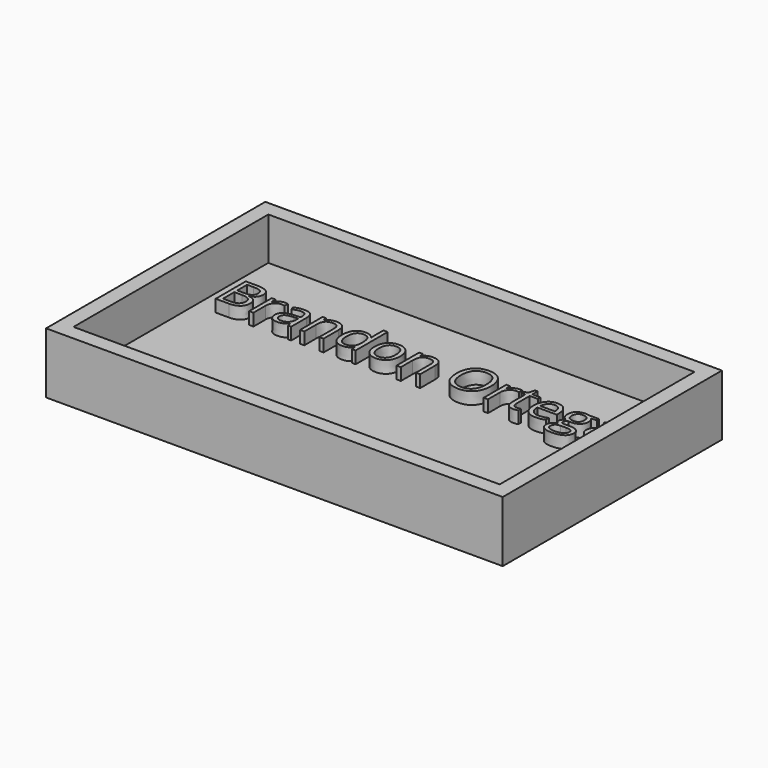
from build123d import *

# Parameters (mm, degrees)
F0_W         = 177.8
F0_H         = 101.6
F1_DEPTH     = 7.62
F0_W_2       = 190.5
F0_H_2       = 114.3
F2_DEPTH     = 25.4
F0_TEXT_SIZE = 21.9972936401
F3_DEPTH     = 12.7


# Not quite as in the source:
# - Text() gives the source's letters only with a copy of the font that has no kerning and outlines rounded to 1/6400 em; it was checked with that copy


with BuildPart() as f1:
    # F0 (on Top) → F1 (new body)
    with BuildSketch(Plane.XY):
        Rectangle(F0_W, F0_H)
        with BuildLine():
            Line((-80.3915155616, 12.7), (-80.3915155616, 28.4040054127))
            Line((-80.3915155616, 28.4040054127), (-75.9542489851, 28.4040054127))
            add(Edge.make_bspline(
                [(-75.9542489851, 28.4040054127), (-72.8299458728, 28.4040054127), (-71.4327740189, 27.469120433)],
                knots=[0, 0, 0, 1, 1, 1], degree=2))
            add(Edge.make_bspline(
                [(-71.4327740189, 27.469120433), (-70.0356021651, 26.5342354533), (-70.0356021651, 24.5166711773)],
                knots=[0, 0, 0, 1, 1, 1], degree=2))
            add(Edge.make_bspline(
                [(-70.0356021651, 24.5166711773), (-70.0356021651, 23.1177807848), (-70.8141001353, 22.2103924222)],
                knots=[0, 0, 0, 1, 1, 1], degree=2))
            add(Edge.make_bspline(
                [(-70.8141001353, 22.2103924222), (-71.5925981055, 21.3030040595), (-73.0877266576, 21.0349120433)],
                knots=[0, 0, 0, 1, 1, 1], degree=2))
            Line((-73.0877266576, 21.0349120433), (-73.0877266576, 20.9283626522))
            add(Edge.make_bspline(
                [(-73.0877266576, 20.9283626522), (-69.509729364, 20.3165629229), (-69.509729364, 17.1682002706)],
                knots=[0, 0, 0, 1, 1, 1], degree=2))
            add(Edge.make_bspline(
                [(-69.509729364, 17.1682002706), (-69.509729364, 15.0647090663), (-70.9326792963, 13.8823545332)],
                knots=[0, 0, 0, 1, 1, 1], degree=2))
            add(Edge.make_bspline(
                [(-70.9326792963, 13.8823545332), (-72.3556292287, 12.7), (-74.9128146143, 12.7)],
                knots=[0, 0, 0, 1, 1, 1], degree=2))
            Line((-74.9128146143, 12.7), (-80.3915155616, 12.7))
        make_face(mode=Mode.SUBTRACT)
        with BuildLine():
            add(Edge.make_bspline(
                [(-63.0652097429, 24.0646955345), (-62.1406359946, 24.6885250338), (-61.0338971583, 24.6885250338)],
                knots=[0, 0, 0, 1, 1, 1], degree=2))
            add(Edge.make_bspline(
                [(-61.0338971583, 24.6885250338), (-60.2502435724, 24.6885250338), (-59.6281326116, 24.5579161028)],
                knots=[0, 0, 0, 1, 1, 1], degree=2))
            Line((-59.6281326116, 24.5579161028), (-59.8756021651, 22.9046820027))
            add(Edge.make_bspline(
                [(-59.8756021651, 22.9046820027), (-60.6042625169, 23.0662246279), (-61.1645060893, 23.0662246279)],
                knots=[0, 0, 0, 1, 1, 1], degree=2))
            add(Edge.make_bspline(
                [(-61.1645060893, 23.0662246279), (-62.5943301759, 23.0662246279), (-63.6082679296, 21.9062110961)],
                knots=[0, 0, 0, 1, 1, 1], degree=2))
            add(Edge.make_bspline(
                [(-63.6082679296, 21.9062110961), (-64.6222056834, 20.7461975643), (-64.6222056834, 19.0173477673)],
                knots=[0, 0, 0, 1, 1, 1], degree=2))
            Line((-64.6222056834, 19.0173477673), (-64.6222056834, 12.7))
            Line((-64.6222056834, 12.7), (-66.4060487145, 12.7))
            Line((-66.4060487145, 12.7), (-66.4060487145, 24.4719891746))
            Line((-66.4060487145, 24.4719891746), (-64.9349797023, 24.4719891746))
            Line((-64.9349797023, 24.4719891746), (-64.7287550744, 22.2928822733))
            Line((-64.7287550744, 22.2928822733), (-64.6428281461, 22.2928822733))
            add(Edge.make_bspline(
                [(-64.6428281461, 22.2928822733), (-63.9897834912, 23.4408660352), (-63.0652097429, 24.0646955345)],
                knots=[0, 0, 0, 1, 1, 1], degree=2))
        make_face(mode=Mode.SUBTRACT)
        with BuildLine():
            Line((-48.8632070365, 12.7), (-50.1864817321, 12.7))
            Line((-50.1864817321, 12.7), (-50.5405006766, 14.3772936401))
            Line((-50.5405006766, 14.3772936401), (-50.6264276049, 14.3772936401))
            add(Edge.make_bspline(
                [(-50.6264276049, 14.3772936401), (-51.5063193505, 13.2705548038), (-52.3810554804, 12.8770094723)],
                knots=[0, 0, 0, 1, 1, 1], degree=2))
            add(Edge.make_bspline(
                [(-52.3810554804, 12.8770094723), (-53.2557916103, 12.4834641407), (-54.5687550744, 12.4834641407)],
                knots=[0, 0, 0, 1, 1, 1], degree=2))
            add(Edge.make_bspline(
                [(-54.5687550744, 12.4834641407), (-56.3182273342, 12.4834641407), (-57.3115426252, 13.3874154263)],
                knots=[0, 0, 0, 1, 1, 1], degree=2))
            add(Edge.make_bspline(
                [(-57.3115426252, 13.3874154263), (-58.3048579161, 14.2913667118), (-58.3048579161, 15.9549120433)],
                knots=[0, 0, 0, 1, 1, 1], degree=2))
            add(Edge.make_bspline(
                [(-58.3048579161, 15.9549120433), (-58.3048579161, 19.5191610284), (-52.6027469553, 19.691014885)],
                knots=[0, 0, 0, 1, 1, 1], degree=2))
            Line((-52.6027469553, 19.691014885), (-50.6058051421, 19.7563193505))
            Line((-50.6058051421, 19.7563193505), (-50.6058051421, 20.4884167794))
            add(Edge.make_bspline(
                [(-50.6058051421, 20.4884167794), (-50.6058051421, 21.8735588633), (-51.2004194858, 22.5334776725)],
                knots=[0, 0, 0, 1, 1, 1], degree=2))
            add(Edge.make_bspline(
                [(-51.2004194858, 22.5334776725), (-51.7950338295, 23.1933964817), (-53.1079972936, 23.1933964817)],
                knots=[0, 0, 0, 1, 1, 1], degree=2))
            add(Edge.make_bspline(
                [(-53.1079972936, 23.1933964817), (-54.5790663058, 23.1933964817), (-56.4350879567, 22.2928822733)],
                knots=[0, 0, 0, 1, 1, 1], degree=2))
            Line((-56.4350879567, 22.2928822733), (-56.9850202977, 23.6574018945))
            add(Edge.make_bspline(
                [(-56.9850202977, 23.6574018945), (-56.1154397835, 24.1282814614), (-55.0791610284, 24.3963734777)],
                knots=[0, 0, 0, 1, 1, 1], degree=2))
            add(Edge.make_bspline(
                [(-55.0791610284, 24.3963734777), (-54.0428822733, 24.6644654939), (-52.9980108254, 24.6644654939)],
                knots=[0, 0, 0, 1, 1, 1], degree=2))
            add(Edge.make_bspline(
                [(-52.9980108254, 24.6644654939), (-50.8945196211, 24.6644654939), (-49.8788633288, 23.7312990528)],
                knots=[0, 0, 0, 1, 1, 1], degree=2))
            add(Edge.make_bspline(
                [(-49.8788633288, 23.7312990528), (-48.8632070365, 22.7981326116), (-48.8632070365, 20.7358863329)],
                knots=[0, 0, 0, 1, 1, 1], degree=2))
            Line((-48.8632070365, 20.7358863329), (-48.8632070365, 12.7))
        make_face(mode=Mode.SUBTRACT)
        with BuildLine():
            Line((-35.3520568336, 12.7), (-37.1358998647, 12.7))
            Line((-37.1358998647, 12.7), (-37.1358998647, 20.3165629229))
            add(Edge.make_bspline(
                [(-37.1358998647, 20.3165629229), (-37.1358998647, 21.7532611637), (-37.7906630582, 22.4630175913)],
                knots=[0, 0, 0, 1, 1, 1], degree=2))
            add(Edge.make_bspline(
                [(-37.7906630582, 22.4630175913), (-38.4454262517, 23.1727740189), (-39.8443166441, 23.1727740189)],
                knots=[0, 0, 0, 1, 1, 1], degree=2))
            add(Edge.make_bspline(
                [(-39.8443166441, 23.1727740189), (-41.6900270636, 23.1727740189), (-42.5492963464, 22.1743031123)],
                knots=[0, 0, 0, 1, 1, 1], degree=2))
            add(Edge.make_bspline(
                [(-42.5492963464, 22.1743031123), (-43.4085656292, 21.1758322057), (-43.4085656292, 18.8764276049)],
                knots=[0, 0, 0, 1, 1, 1], degree=2))
            Line((-43.4085656292, 18.8764276049), (-43.4085656292, 12.7))
            Line((-43.4085656292, 12.7), (-45.1924086604, 12.7))
            Line((-45.1924086604, 12.7), (-45.1924086604, 24.4719891746))
            Line((-45.1924086604, 24.4719891746), (-43.741962111, 24.4719891746))
            Line((-43.741962111, 24.4719891746), (-43.4532476319, 22.86))
            Line((-43.4532476319, 22.86), (-43.3673207037, 22.86))
            add(Edge.make_bspline(
                [(-43.3673207037, 22.86), (-42.8173883627, 23.7295805142), (-41.8292286874, 24.209052774)],
                knots=[0, 0, 0, 1, 1, 1], degree=2))
            add(Edge.make_bspline(
                [(-41.8292286874, 24.209052774), (-40.8410690122, 24.6885250338), (-39.6277807848, 24.6885250338)],
                knots=[0, 0, 0, 1, 1, 1], degree=2))
            add(Edge.make_bspline(
                [(-39.6277807848, 24.6885250338), (-37.5002300406, 24.6885250338), (-36.4261434371, 23.6625575101)],
                knots=[0, 0, 0, 1, 1, 1], degree=2))
            add(Edge.make_bspline(
                [(-36.4261434371, 23.6625575101), (-35.3520568336, 22.6365899865), (-35.3520568336, 20.3784303112)],
                knots=[0, 0, 0, 1, 1, 1], degree=2))
            Line((-35.3520568336, 20.3784303112), (-35.3520568336, 12.7))
        make_face(mode=Mode.SUBTRACT)
        with BuildLine():
            Line((-23.4425845737, 12.7), (-23.6797428958, 14.2776184032))
            Line((-23.6797428958, 14.2776184032), (-23.7759810555, 14.2776184032))
            add(Edge.make_bspline(
                [(-23.7759810555, 14.2776184032), (-25.0098917456, 12.4834641407), (-27.4708389716, 12.4834641407)],
                knots=[0, 0, 0, 1, 1, 1], degree=2))
            add(Edge.make_bspline(
                [(-27.4708389716, 12.4834641407), (-29.7805548038, 12.4834641407), (-31.0643031123, 14.0628010825)],
                knots=[0, 0, 0, 1, 1, 1], degree=2))
            add(Edge.make_bspline(
                [(-31.0643031123, 14.0628010825), (-32.3480514208, 15.6421380244), (-32.3480514208, 18.5533423545)],
                knots=[0, 0, 0, 1, 1, 1], degree=2))
            add(Edge.make_bspline(
                [(-32.3480514208, 18.5533423545), (-32.3480514208, 21.4645466847), (-31.0591474966, 23.0765358593)],
                knots=[0, 0, 0, 1, 1, 1], degree=2))
            add(Edge.make_bspline(
                [(-31.0591474966, 23.0765358593), (-29.7702435724, 24.6885250338), (-27.4708389716, 24.6885250338)],
                knots=[0, 0, 0, 1, 1, 1], degree=2))
            add(Edge.make_bspline(
                [(-27.4708389716, 24.6885250338), (-25.0751962111, 24.6885250338), (-23.7966035183, 22.9459269283)],
                knots=[0, 0, 0, 1, 1, 1], degree=2))
            Line((-23.7966035183, 22.9459269283), (-23.6556833559, 22.9459269283))
            Line((-23.6556833559, 22.9459269283), (-23.7312990528, 23.7948849797))
            Line((-23.7312990528, 23.7948849797), (-23.7759810555, 24.6232205683))
            Line((-23.7759810555, 24.6232205683), (-23.7759810555, 29.4145060893))
            Line((-23.7759810555, 29.4145060893), (-21.9921380244, 29.4145060893))
            Line((-21.9921380244, 29.4145060893), (-21.9921380244, 12.7))
            Line((-21.9921380244, 12.7), (-23.4425845737, 12.7))
        make_face(mode=Mode.SUBTRACT)
        with BuildLine():
            add(Edge.make_bspline(
                [(-9.5069553451, 23.0438836265), (-8.05135318, 21.3992422192), (-8.05135318, 18.5980243572)],
                knots=[0, 0, 0, 1, 1, 1], degree=2))
            add(Edge.make_bspline(
                [(-8.05135318, 18.5980243572), (-8.05135318, 15.7177537212), (-9.5000811908, 14.100608931)],
                knots=[0, 0, 0, 1, 1, 1], degree=2))
            add(Edge.make_bspline(
                [(-9.5000811908, 14.100608931), (-10.9488092016, 12.4834641407), (-13.5059945873, 12.4834641407)],
                knots=[0, 0, 0, 1, 1, 1], degree=2))
            add(Edge.make_bspline(
                [(-13.5059945873, 12.4834641407), (-15.0870500677, 12.4834641407), (-16.3106495264, 13.2258728011)],
                knots=[0, 0, 0, 1, 1, 1], degree=2))
            add(Edge.make_bspline(
                [(-16.3106495264, 13.2258728011), (-17.5342489851, 13.9682814614), (-18.2010419486, 15.3534235453)],
                knots=[0, 0, 0, 1, 1, 1], degree=2))
            add(Edge.make_bspline(
                [(-18.2010419486, 15.3534235453), (-18.867834912, 16.7385656292), (-18.867834912, 18.5980243572)],
                knots=[0, 0, 0, 1, 1, 1], degree=2))
            add(Edge.make_bspline(
                [(-18.867834912, 18.5980243572), (-18.867834912, 21.4748579161), (-17.427699594, 23.081691475)],
                knots=[0, 0, 0, 1, 1, 1], degree=2))
            add(Edge.make_bspline(
                [(-17.427699594, 23.081691475), (-15.987564276, 24.6885250338), (-13.4303788904, 24.6885250338)],
                knots=[0, 0, 0, 1, 1, 1], degree=2))
            add(Edge.make_bspline(
                [(-13.4303788904, 24.6885250338), (-10.9625575101, 24.6885250338), (-9.5069553451, 23.0438836265)],
                knots=[0, 0, 0, 1, 1, 1], degree=2))
        make_face(mode=Mode.SUBTRACT)
        with BuildLine():
            Line((4.9167388363, 12.7), (3.1328958051, 12.7))
            Line((3.1328958051, 12.7), (3.1328958051, 20.3165629229))
            add(Edge.make_bspline(
                [(3.1328958051, 20.3165629229), (3.1328958051, 21.7532611637), (2.4781326116, 22.4630175913)],
                knots=[0, 0, 0, 1, 1, 1], degree=2))
            add(Edge.make_bspline(
                [(2.4781326116, 22.4630175913), (1.8233694181, 23.1727740189), (0.4244790257, 23.1727740189)],
                knots=[0, 0, 0, 1, 1, 1], degree=2))
            add(Edge.make_bspline(
                [(0.4244790257, 23.1727740189), (-1.4212313938, 23.1727740189), (-2.2805006766, 22.1743031123)],
                knots=[0, 0, 0, 1, 1, 1], degree=2))
            add(Edge.make_bspline(
                [(-2.2805006766, 22.1743031123), (-3.1397699594, 21.1758322057), (-3.1397699594, 18.8764276049)],
                knots=[0, 0, 0, 1, 1, 1], degree=2))
            Line((-3.1397699594, 18.8764276049), (-3.1397699594, 12.7))
            Line((-3.1397699594, 12.7), (-4.9236129905, 12.7))
            Line((-4.9236129905, 12.7), (-4.9236129905, 24.4719891746))
            Line((-4.9236129905, 24.4719891746), (-3.4731664411, 24.4719891746))
            Line((-3.4731664411, 24.4719891746), (-3.1844519621, 22.86))
            Line((-3.1844519621, 22.86), (-3.0985250338, 22.86))
            add(Edge.make_bspline(
                [(-3.0985250338, 22.86), (-2.5485926928, 23.7295805142), (-1.5604330176, 24.209052774)],
                knots=[0, 0, 0, 1, 1, 1], degree=2))
            add(Edge.make_bspline(
                [(-1.5604330176, 24.209052774), (-0.5722733424, 24.6885250338), (0.641014885, 24.6885250338)],
                knots=[0, 0, 0, 1, 1, 1], degree=2))
            add(Edge.make_bspline(
                [(0.641014885, 24.6885250338), (2.7685656292, 24.6885250338), (3.8426522327, 23.6625575101)],
                knots=[0, 0, 0, 1, 1, 1], degree=2))
            add(Edge.make_bspline(
                [(3.8426522327, 23.6625575101), (4.9167388363, 22.6365899865), (4.9167388363, 20.3784303112)],
                knots=[0, 0, 0, 1, 1, 1], degree=2))
            Line((4.9167388363, 20.3784303112), (4.9167388363, 12.7))
        make_face(mode=Mode.SUBTRACT)
        with BuildLine():
            add(Edge.make_bspline(
                [(26.2919215156, 26.5033017591), (28.1926251691, 24.3551285521), (28.1926251691, 20.5743437077)],
                knots=[0, 0, 0, 1, 1, 1], degree=2))
            add(Edge.make_bspline(
                [(28.1926251691, 20.5743437077), (28.1926251691, 16.8038700947), (26.2850473613, 14.6436671177)],
                knots=[0, 0, 0, 1, 1, 1], degree=2))
            add(Edge.make_bspline(
                [(26.2850473613, 14.6436671177), (24.3774695535, 12.4834641407), (20.9850744249, 12.4834641407)],
                knots=[0, 0, 0, 1, 1, 1], degree=2))
            add(Edge.make_bspline(
                [(20.9850744249, 12.4834641407), (17.5170635995, 12.4834641407), (15.631826793, 14.6058592693)],
                knots=[0, 0, 0, 1, 1, 1], degree=2))
            add(Edge.make_bspline(
                [(15.631826793, 14.6058592693), (13.7465899865, 16.7282543978), (13.7465899865, 20.5949661705)],
                knots=[0, 0, 0, 1, 1, 1], degree=2))
            add(Edge.make_bspline(
                [(13.7465899865, 20.5949661705), (13.7465899865, 24.430744249), (15.6369824087, 26.5411096076)],
                knots=[0, 0, 0, 1, 1, 1], degree=2))
            add(Edge.make_bspline(
                [(15.6369824087, 26.5411096076), (17.5273748309, 28.6514749662), (21.0056968877, 28.6514749662)],
                knots=[0, 0, 0, 1, 1, 1], degree=2))
            add(Edge.make_bspline(
                [(21.0056968877, 28.6514749662), (24.391217862, 28.6514749662), (26.2919215156, 26.5033017591)],
                knots=[0, 0, 0, 1, 1, 1], degree=2))
        make_face(mode=Mode.SUBTRACT)
        with BuildLine():
            add(Edge.make_bspline(
                [(34.7643166441, 24.0646955345), (35.6888903924, 24.6885250338), (36.7956292287, 24.6885250338)],
                knots=[0, 0, 0, 1, 1, 1], degree=2))
            add(Edge.make_bspline(
                [(36.7956292287, 24.6885250338), (37.5792828146, 24.6885250338), (38.2013937754, 24.5579161028)],
                knots=[0, 0, 0, 1, 1, 1], degree=2))
            Line((38.2013937754, 24.5579161028), (37.9539242219, 22.9046820027))
            add(Edge.make_bspline(
                [(37.9539242219, 22.9046820027), (37.2252638701, 23.0662246279), (36.6650202977, 23.0662246279)],
                knots=[0, 0, 0, 1, 1, 1], degree=2))
            add(Edge.make_bspline(
                [(36.6650202977, 23.0662246279), (35.2351962111, 23.0662246279), (34.2212584574, 21.9062110961)],
                knots=[0, 0, 0, 1, 1, 1], degree=2))
            add(Edge.make_bspline(
                [(34.2212584574, 21.9062110961), (33.2073207037, 20.7461975643), (33.2073207037, 19.0173477673)],
                knots=[0, 0, 0, 1, 1, 1], degree=2))
            Line((33.2073207037, 19.0173477673), (33.2073207037, 12.7))
            Line((33.2073207037, 12.7), (31.4234776725, 12.7))
            Line((31.4234776725, 12.7), (31.4234776725, 24.4719891746))
            Line((31.4234776725, 24.4719891746), (32.8945466847, 24.4719891746))
            Line((32.8945466847, 24.4719891746), (33.1007713126, 22.2928822733))
            Line((33.1007713126, 22.2928822733), (33.1866982409, 22.2928822733))
            add(Edge.make_bspline(
                [(33.1866982409, 22.2928822733), (33.8397428958, 23.4408660352), (34.7643166441, 24.0646955345)],
                knots=[0, 0, 0, 1, 1, 1], degree=2))
        make_face(mode=Mode.SUBTRACT)
        with BuildLine():
            add(Edge.make_bspline(
                [(42.8208254398, 14.5268064953), (43.3260757781, 13.95797023), (44.2059675237, 13.95797023)],
                knots=[0, 0, 0, 1, 1, 1], degree=2))
            add(Edge.make_bspline(
                [(44.2059675237, 13.95797023), (44.6802841678, 13.95797023), (45.1202300406, 14.0267117727)],
                knots=[0, 0, 0, 1, 1, 1], degree=2))
            add(Edge.make_bspline(
                [(45.1202300406, 14.0267117727), (45.5601759134, 14.0954533153), (45.8179566982, 14.1710690122)],
                knots=[0, 0, 0, 1, 1, 1], degree=2))
            Line((45.8179566982, 14.1710690122), (45.8179566982, 12.8065493911))
            add(Edge.make_bspline(
                [(45.8179566982, 12.8065493911), (45.5292422192, 12.6690663058), (44.9655615697, 12.5762652233)],
                knots=[0, 0, 0, 1, 1, 1], degree=2))
            add(Edge.make_bspline(
                [(44.9655615697, 12.5762652233), (44.4018809202, 12.4834641407), (43.9481867388, 12.4834641407)],
                knots=[0, 0, 0, 1, 1, 1], degree=2))
            add(Edge.make_bspline(
                [(43.9481867388, 12.4834641407), (40.5351691475, 12.4834641407), (40.5351691475, 16.0820838972)],
                knots=[0, 0, 0, 1, 1, 1], degree=2))
            Line((40.5351691475, 16.0820838972), (40.5351691475, 23.0868470907))
            Line((40.5351691475, 23.0868470907), (38.847564276, 23.0868470907))
            Line((38.847564276, 23.0868470907), (38.847564276, 23.9461163735))
            Line((38.847564276, 23.9461163735), (40.5351691475, 24.6885250338))
            Line((40.5351691475, 24.6885250338), (41.2844519621, 27.2010284168))
            Line((41.2844519621, 27.2010284168), (42.3155751015, 27.2010284168))
            Line((42.3155751015, 27.2010284168), (42.3155751015, 24.4719891746))
            Line((42.3155751015, 24.4719891746), (45.73202977, 24.4719891746))
            Line((45.73202977, 24.4719891746), (45.73202977, 23.0868470907))
            Line((45.73202977, 23.0868470907), (42.3155751015, 23.0868470907))
            Line((42.3155751015, 23.0868470907), (42.3155751015, 16.157699594))
            add(Edge.make_bspline(
                [(42.3155751015, 16.157699594), (42.3155751015, 15.0956427605), (42.8208254398, 14.5268064953)],
                knots=[0, 0, 0, 1, 1, 1], degree=2))
        make_face(mode=Mode.SUBTRACT)
        with BuildLine():
            add(Edge.make_bspline(
                [(55.1771177267, 12.6621921516), (54.3350338295, 12.4834641407), (53.142368065, 12.4834641407)],
                knots=[0, 0, 0, 1, 1, 1], degree=2))
            add(Edge.make_bspline(
                [(53.142368065, 12.4834641407), (50.5336265223, 12.4834641407), (49.0230311231, 14.0748308525)],
                knots=[0, 0, 0, 1, 1, 1], degree=2))
            add(Edge.make_bspline(
                [(49.0230311231, 14.0748308525), (47.512435724, 15.6661975643), (47.512435724, 18.488037889)],
                knots=[0, 0, 0, 1, 1, 1], degree=2))
            add(Edge.make_bspline(
                [(47.512435724, 18.488037889), (47.512435724, 21.3373748309), (48.9147631935, 23.0129499323)],
                knots=[0, 0, 0, 1, 1, 1], degree=2))
            add(Edge.make_bspline(
                [(48.9147631935, 23.0129499323), (50.3170906631, 24.6885250338), (52.6817997294, 24.6885250338)],
                knots=[0, 0, 0, 1, 1, 1], degree=2))
            add(Edge.make_bspline(
                [(52.6817997294, 24.6885250338), (54.8918403248, 24.6885250338), (56.180744249, 23.2329228687)],
                knots=[0, 0, 0, 1, 1, 1], degree=2))
            add(Edge.make_bspline(
                [(56.180744249, 23.2329228687), (57.4696481732, 21.7773207037), (57.4696481732, 19.3919891746)],
                knots=[0, 0, 0, 1, 1, 1], degree=2))
            Line((57.4696481732, 19.3919891746), (57.4696481732, 18.2646278755))
            Line((57.4696481732, 18.2646278755), (49.3615832206, 18.2646278755))
            add(Edge.make_bspline(
                [(49.3615832206, 18.2646278755), (49.4165764547, 16.1920703654), (50.4098917456, 15.1179837618)],
                knots=[0, 0, 0, 1, 1, 1], degree=2))
            add(Edge.make_bspline(
                [(50.4098917456, 15.1179837618), (51.4032070365, 14.0438971583), (53.2076725304, 14.0438971583)],
                knots=[0, 0, 0, 1, 1, 1], degree=2))
            add(Edge.make_bspline(
                [(53.2076725304, 14.0438971583), (55.108376184, 14.0438971583), (56.9643978349, 14.8378619756)],
                knots=[0, 0, 0, 1, 1, 1], degree=2))
            Line((56.9643978349, 14.8378619756), (56.9643978349, 13.2464952639))
            add(Edge.make_bspline(
                [(56.9643978349, 13.2464952639), (56.0192016238, 12.8409201624), (55.1771177267, 12.6621921516)],
                knots=[0, 0, 0, 1, 1, 1], degree=2))
        make_face(mode=Mode.SUBTRACT)
        with BuildLine():
            Line((66.0760893099, 24.4719891746), (70.1455886333, 24.4719891746))
            Line((70.1455886333, 24.4719891746), (70.1455886333, 23.3446278755))
            Line((70.1455886333, 23.3446278755), (67.9664817321, 23.0868470907))
            add(Edge.make_bspline(
                [(67.9664817321, 23.0868470907), (68.2655074425, 22.7122056834), (68.5026657645, 22.1038430311)],
                knots=[0, 0, 0, 1, 1, 1], degree=2))
            add(Edge.make_bspline(
                [(68.5026657645, 22.1038430311), (68.7398240866, 21.4954803789), (68.7398240866, 20.7358863329)],
                knots=[0, 0, 0, 1, 1, 1], degree=2))
            add(Edge.make_bspline(
                [(68.7398240866, 20.7358863329), (68.7398240866, 19.0035994587), (67.5574695535, 17.9724763194)],
                knots=[0, 0, 0, 1, 1, 1], degree=2))
            add(Edge.make_bspline(
                [(67.5574695535, 17.9724763194), (66.3751150203, 16.94135318), (64.3128687415, 16.94135318)],
                knots=[0, 0, 0, 1, 1, 1], degree=2))
            add(Edge.make_bspline(
                [(64.3128687415, 16.94135318), (63.7869959405, 16.94135318), (63.3264276049, 17.0272801083)],
                knots=[0, 0, 0, 1, 1, 1], degree=2))
            add(Edge.make_bspline(
                [(63.3264276049, 17.0272801083), (62.1887550744, 16.4257916103), (62.1887550744, 15.5149661705)],
                knots=[0, 0, 0, 1, 1, 1], degree=2))
            add(Edge.make_bspline(
                [(62.1887550744, 15.5149661705), (62.1887550744, 15.030338295), (62.5857374831, 14.8000541272)],
                knots=[0, 0, 0, 1, 1, 1], degree=2))
            add(Edge.make_bspline(
                [(62.5857374831, 14.8000541272), (62.9827198917, 14.5697699594), (63.9485385656, 14.5697699594)],
                knots=[0, 0, 0, 1, 1, 1], degree=2))
            Line((63.9485385656, 14.5697699594), (66.0314073072, 14.5697699594))
            add(Edge.make_bspline(
                [(66.0314073072, 14.5697699594), (67.9458592693, 14.5697699594), (68.9701082544, 13.7637753721)],
                knots=[0, 0, 0, 1, 1, 1], degree=2))
            add(Edge.make_bspline(
                [(68.9701082544, 13.7637753721), (69.9943572395, 12.9577807848), (69.9943572395, 11.4214073072)],
                knots=[0, 0, 0, 1, 1, 1], degree=2))
            add(Edge.make_bspline(
                [(69.9943572395, 11.4214073072), (69.9943572395, 9.4657104195), (68.4270500677, 8.4397428958)],
                knots=[0, 0, 0, 1, 1, 1], degree=2))
            add(Edge.make_bspline(
                [(68.4270500677, 8.4397428958), (66.8597428958, 7.4137753721), (63.852300406, 7.4137753721)],
                knots=[0, 0, 0, 1, 1, 1], degree=2))
            add(Edge.make_bspline(
                [(63.852300406, 7.4137753721), (61.5425845737, 7.4137753721), (60.291488498, 8.2730446549)],
                knots=[0, 0, 0, 1, 1, 1], degree=2))
            add(Edge.make_bspline(
                [(60.291488498, 8.2730446549), (59.0403924222, 9.1323139378), (59.0403924222, 10.7030581867)],
                knots=[0, 0, 0, 1, 1, 1], degree=2))
            add(Edge.make_bspline(
                [(59.0403924222, 10.7030581867), (59.0403924222, 11.7754262517), (59.7278078484, 12.5607983762)],
                knots=[0, 0, 0, 1, 1, 1], degree=2))
            add(Edge.make_bspline(
                [(59.7278078484, 12.5607983762), (60.4152232747, 13.3461705007), (61.6594451962, 13.6245737483)],
                knots=[0, 0, 0, 1, 1, 1], degree=2))
            add(Edge.make_bspline(
                [(61.6594451962, 13.6245737483), (61.209188092, 13.8273612991), (60.9032882273, 14.2569959405)],
                knots=[0, 0, 0, 1, 1, 1], degree=2))
            add(Edge.make_bspline(
                [(60.9032882273, 14.2569959405), (60.5973883627, 14.6866305819), (60.5973883627, 15.2571853857)],
                knots=[0, 0, 0, 1, 1, 1], degree=2))
            add(Edge.make_bspline(
                [(60.5973883627, 15.2571853857), (60.5973883627, 15.8999188092), (60.9410960758, 16.3845466847)],
                knots=[0, 0, 0, 1, 1, 1], degree=2))
            add(Edge.make_bspline(
                [(60.9410960758, 16.3845466847), (61.2848037889, 16.8691745602), (62.0272124493, 17.3194316644)],
                knots=[0, 0, 0, 1, 1, 1], degree=2))
            add(Edge.make_bspline(
                [(62.0272124493, 17.3194316644), (61.1129499323, 17.6940730717), (60.5389580514, 18.5963058187)],
                knots=[0, 0, 0, 1, 1, 1], degree=2))
            add(Edge.make_bspline(
                [(60.5389580514, 18.5963058187), (59.9649661705, 19.4985385656), (59.9649661705, 20.660270636)],
                knots=[0, 0, 0, 1, 1, 1], degree=2))
            add(Edge.make_bspline(
                [(59.9649661705, 20.660270636), (59.9649661705, 22.5919079838), (61.1249797023, 23.6402165088)],
                knots=[0, 0, 0, 1, 1, 1], degree=2))
            add(Edge.make_bspline(
                [(61.1249797023, 23.6402165088), (62.2849932341, 24.6885250338), (64.4091069012, 24.6885250338)],
                knots=[0, 0, 0, 1, 1, 1], degree=2))
            add(Edge.make_bspline(
                [(64.4091069012, 24.6885250338), (65.3336806495, 24.6885250338), (66.0760893099, 24.4719891746)],
                knots=[0, 0, 0, 1, 1, 1], degree=2))
        make_face(mode=Mode.SUBTRACT)
        with BuildLine():
            Line((81.1236129905, 12.7), (79.800338295, 12.7))
            Line((79.800338295, 12.7), (79.4463193505, 14.3772936401))
            Line((79.4463193505, 14.3772936401), (79.3603924222, 14.3772936401))
            add(Edge.make_bspline(
                [(79.3603924222, 14.3772936401), (78.4805006766, 13.2705548038), (77.6057645467, 12.8770094723)],
                knots=[0, 0, 0, 1, 1, 1], degree=2))
            add(Edge.make_bspline(
                [(77.6057645467, 12.8770094723), (76.7310284168, 12.4834641407), (75.4180649526, 12.4834641407)],
                knots=[0, 0, 0, 1, 1, 1], degree=2))
            add(Edge.make_bspline(
                [(75.4180649526, 12.4834641407), (73.6685926928, 12.4834641407), (72.6752774019, 13.3874154263)],
                knots=[0, 0, 0, 1, 1, 1], degree=2))
            add(Edge.make_bspline(
                [(72.6752774019, 13.3874154263), (71.681962111, 14.2913667118), (71.681962111, 15.9549120433)],
                knots=[0, 0, 0, 1, 1, 1], degree=2))
            add(Edge.make_bspline(
                [(71.681962111, 15.9549120433), (71.681962111, 19.5191610284), (77.3840730717, 19.691014885)],
                knots=[0, 0, 0, 1, 1, 1], degree=2))
            Line((77.3840730717, 19.691014885), (79.381014885, 19.7563193505))
            Line((79.381014885, 19.7563193505), (79.381014885, 20.4884167794))
            add(Edge.make_bspline(
                [(79.381014885, 20.4884167794), (79.381014885, 21.8735588633), (78.7864005413, 22.5334776725)],
                knots=[0, 0, 0, 1, 1, 1], degree=2))
            add(Edge.make_bspline(
                [(78.7864005413, 22.5334776725), (78.1917861976, 23.1933964817), (76.8788227334, 23.1933964817)],
                knots=[0, 0, 0, 1, 1, 1], degree=2))
            add(Edge.make_bspline(
                [(76.8788227334, 23.1933964817), (75.4077537212, 23.1933964817), (73.5517320704, 22.2928822733)],
                knots=[0, 0, 0, 1, 1, 1], degree=2))
            Line((73.5517320704, 22.2928822733), (73.0017997294, 23.6574018945))
            add(Edge.make_bspline(
                [(73.0017997294, 23.6574018945), (73.8713802436, 24.1282814614), (74.9076589986, 24.3963734777)],
                knots=[0, 0, 0, 1, 1, 1], degree=2))
            add(Edge.make_bspline(
                [(74.9076589986, 24.3963734777), (75.9439377537, 24.6644654939), (76.9888092016, 24.6644654939)],
                knots=[0, 0, 0, 1, 1, 1], degree=2))
            add(Edge.make_bspline(
                [(76.9888092016, 24.6644654939), (79.092300406, 24.6644654939), (80.1079566982, 23.7312990528)],
                knots=[0, 0, 0, 1, 1, 1], degree=2))
            add(Edge.make_bspline(
                [(80.1079566982, 23.7312990528), (81.1236129905, 22.7981326116), (81.1236129905, 20.7358863329)],
                knots=[0, 0, 0, 1, 1, 1], degree=2))
            Line((81.1236129905, 20.7358863329), (81.1236129905, 12.7))
        make_face(mode=Mode.SUBTRACT)
    extrude(amount=F1_DEPTH)

    # F0 (on Top) → F2 (join)
    with BuildSketch(Plane.XY):
        Rectangle(F0_W_2, F0_H_2)
        Rectangle(F0_W, F0_H, mode=Mode.SUBTRACT)
    extrude(amount=F2_DEPTH)



with BuildPart() as f1b:
    # F0 (on Top) → F1, piece 2 (new body)
    with BuildSketch(Plane.XY):
        with BuildLine():
            Line((-78.5664276049, 26.8229499323), (-78.5664276049, 21.681082544))
            Line((-78.5664276049, 21.681082544), (-75.558985115, 21.681082544))
            add(Edge.make_bspline(
                [(-75.558985115, 21.681082544), (-73.6239106901, 21.681082544), (-72.7749526387, 22.2877266576)],
                knots=[0, 0, 0, 1, 1, 1], degree=2))
            add(Edge.make_bspline(
                [(-72.7749526387, 22.2877266576), (-71.9259945873, 22.8943707713), (-71.9259945873, 24.3310690122)],
                knots=[0, 0, 0, 1, 1, 1], degree=2))
            add(Edge.make_bspline(
                [(-71.9259945873, 24.3310690122), (-71.9259945873, 25.6543437077), (-72.8711907984, 26.23864682)],
                knots=[0, 0, 0, 1, 1, 1], degree=2))
            add(Edge.make_bspline(
                [(-72.8711907984, 26.23864682), (-73.8163870095, 26.8229499323), (-75.8786332882, 26.8229499323)],
                knots=[0, 0, 0, 1, 1, 1], degree=2))
            Line((-75.8786332882, 26.8229499323), (-78.5664276049, 26.8229499323))
        make_face()
    extrude(amount=F1_DEPTH)


with BuildPart() as f1c:
    # F0 (on Top) → F1, piece 3 (new body)
    with BuildSketch(Plane.XY):
        with BuildLine():
            Line((-75.4386874154, 20.1343978349), (-78.5664276049, 20.1343978349))
            Line((-78.5664276049, 20.1343978349), (-78.5664276049, 14.2569959405))
            Line((-78.5664276049, 14.2569959405), (-75.2874560217, 14.2569959405))
            add(Edge.make_bspline(
                [(-75.2874560217, 14.2569959405), (-73.3867523681, 14.2569959405), (-72.4260893099, 14.9925304465)],
                knots=[0, 0, 0, 1, 1, 1], degree=2))
            add(Edge.make_bspline(
                [(-72.4260893099, 14.9925304465), (-71.4654262517, 15.7280649526), (-71.4654262517, 17.2988092016)],
                knots=[0, 0, 0, 1, 1, 1], degree=2))
            add(Edge.make_bspline(
                [(-71.4654262517, 17.2988092016), (-71.4654262517, 18.7595669824), (-72.4484303112, 19.4469824087)],
                knots=[0, 0, 0, 1, 1, 1], degree=2))
            add(Edge.make_bspline(
                [(-72.4484303112, 19.4469824087), (-73.4314343708, 20.1343978349), (-75.4386874154, 20.1343978349)],
                knots=[0, 0, 0, 1, 1, 1], degree=2))
        make_face()
    extrude(amount=F1_DEPTH)


with BuildPart() as f1d:
    # F0 (on Top) → F1, piece 4 (new body)
    with BuildSketch(Plane.XY):
        with BuildLine():
            add(Edge.make_bspline(
                [(-55.8507848444, 14.4615020298), (-55.2664817321, 13.95797023), (-54.2147361299, 13.95797023)],
                knots=[0, 0, 0, 1, 1, 1], degree=2))
            add(Edge.make_bspline(
                [(-54.2147361299, 13.95797023), (-52.5477537212, 13.95797023), (-51.5974018945, 14.8705142084)],
                knots=[0, 0, 0, 1, 1, 1], degree=2))
            add(Edge.make_bspline(
                [(-51.5974018945, 14.8705142084), (-50.6470500677, 15.7830581867), (-50.6470500677, 17.4259810555)],
                knots=[0, 0, 0, 1, 1, 1], degree=2))
            Line((-50.6470500677, 17.4259810555), (-50.6470500677, 18.488037889))
            Line((-50.6470500677, 18.488037889), (-52.4308930988, 18.4158592693))
            add(Edge.make_bspline(
                [(-52.4308930988, 18.4158592693), (-54.558443843, 18.3402435724), (-55.4967658999, 17.7542219215)],
                knots=[0, 0, 0, 1, 1, 1], degree=2))
            add(Edge.make_bspline(
                [(-55.4967658999, 17.7542219215), (-56.4350879567, 17.1682002706), (-56.4350879567, 15.9342895805)],
                knots=[0, 0, 0, 1, 1, 1], degree=2))
            add(Edge.make_bspline(
                [(-56.4350879567, 15.9342895805), (-56.4350879567, 14.9650338295), (-55.8507848444, 14.4615020298)],
                knots=[0, 0, 0, 1, 1, 1], degree=2))
        make_face()
    extrude(amount=F1_DEPTH)


with BuildPart() as f1e:
    # F0 (on Top) → F1, piece 5 (new body)
    with BuildSketch(Plane.XY):
        with BuildLine():
            add(Edge.make_bspline(
                [(-29.6722868742, 15.1282949932), (-28.8456698241, 13.9785926928), (-27.2439918809, 13.9785926928)],
                knots=[0, 0, 0, 1, 1, 1], degree=2))
            add(Edge.make_bspline(
                [(-27.2439918809, 13.9785926928), (-25.4189039242, 13.9785926928), (-24.5974424899, 14.9719079838)],
                knots=[0, 0, 0, 1, 1, 1], degree=2))
            add(Edge.make_bspline(
                [(-24.5974424899, 14.9719079838), (-23.7759810555, 15.9652232747), (-23.7759810555, 18.1787009472)],
                knots=[0, 0, 0, 1, 1, 1], degree=2))
            Line((-23.7759810555, 18.1787009472), (-23.7759810555, 18.5533423545))
            add(Edge.make_bspline(
                [(-23.7759810555, 18.5533423545), (-23.7759810555, 21.0555345061), (-24.6077537212, 22.1244654939)],
                knots=[0, 0, 0, 1, 1, 1], degree=2))
            add(Edge.make_bspline(
                [(-24.6077537212, 22.1244654939), (-25.439526387, 23.1933964817), (-27.2646143437, 23.1933964817)],
                knots=[0, 0, 0, 1, 1, 1], degree=2))
            add(Edge.make_bspline(
                [(-27.2646143437, 23.1933964817), (-28.8353585927, 23.1933964817), (-29.6671312585, 21.9749526387)],
                knots=[0, 0, 0, 1, 1, 1], degree=2))
            add(Edge.make_bspline(
                [(-29.6671312585, 21.9749526387), (-30.4989039242, 20.7565087957), (-30.4989039242, 18.5327198917)],
                knots=[0, 0, 0, 1, 1, 1], degree=2))
            add(Edge.make_bspline(
                [(-30.4989039242, 18.5327198917), (-30.4989039242, 16.2779972936), (-29.6722868742, 15.1282949932)],
                knots=[0, 0, 0, 1, 1, 1], degree=2))
        make_face()
    extrude(amount=F1_DEPTH)


with BuildPart() as f1f:
    # F0 (on Top) → F1, piece 6 (new body)
    with BuildSketch(Plane.XY):
        with BuildLine():
            add(Edge.make_bspline(
                [(-16.1267658999, 22.0230717185), (-17.0186874154, 20.8733694181), (-17.0186874154, 18.5980243572)],
                knots=[0, 0, 0, 1, 1, 1], degree=2))
            add(Edge.make_bspline(
                [(-17.0186874154, 18.5980243572), (-17.0186874154, 16.339864682), (-16.1164546685, 15.1592286874)],
                knots=[0, 0, 0, 1, 1, 1], degree=2))
            add(Edge.make_bspline(
                [(-16.1164546685, 15.1592286874), (-15.2142219215, 13.9785926928), (-13.4647496617, 13.9785926928)],
                knots=[0, 0, 0, 1, 1, 1], degree=2))
            add(Edge.make_bspline(
                [(-13.4647496617, 13.9785926928), (-11.7118403248, 13.9785926928), (-10.8044519621, 15.1540730717)],
                knots=[0, 0, 0, 1, 1, 1], degree=2))
            add(Edge.make_bspline(
                [(-10.8044519621, 15.1540730717), (-9.8970635995, 16.3295534506), (-9.8970635995, 18.5980243572)],
                knots=[0, 0, 0, 1, 1, 1], degree=2))
            add(Edge.make_bspline(
                [(-9.8970635995, 18.5980243572), (-9.8970635995, 20.842435724), (-10.8044519621, 22.0076048714)],
                knots=[0, 0, 0, 1, 1, 1], degree=2))
            add(Edge.make_bspline(
                [(-10.8044519621, 22.0076048714), (-11.7118403248, 23.1727740189), (-13.4853721245, 23.1727740189)],
                knots=[0, 0, 0, 1, 1, 1], degree=2))
            add(Edge.make_bspline(
                [(-13.4853721245, 23.1727740189), (-15.2348443843, 23.1727740189), (-16.1267658999, 22.0230717185)],
                knots=[0, 0, 0, 1, 1, 1], degree=2))
        make_face()
    extrude(amount=F1_DEPTH)


with BuildPart() as f1g:
    # F0 (on Top) → F1, piece 7 (new body)
    with BuildSketch(Plane.XY):
        with BuildLine():
            add(Edge.make_bspline(
                [(17.0375913396, 25.3690663058), (15.6782273342, 23.7192692828), (15.6782273342, 20.5743437077)],
                knots=[0, 0, 0, 1, 1, 1], degree=2))
            add(Edge.make_bspline(
                [(15.6782273342, 20.5743437077), (15.6782273342, 17.3847361299), (17.0375913396, 15.7349391069)],
                knots=[0, 0, 0, 1, 1, 1], degree=2))
            add(Edge.make_bspline(
                [(17.0375913396, 15.7349391069), (18.3969553451, 14.0851420839), (20.9850744249, 14.0851420839)],
                knots=[0, 0, 0, 1, 1, 1], degree=2))
            add(Edge.make_bspline(
                [(20.9850744249, 14.0851420839), (23.5938159675, 14.0851420839), (24.9256833559, 15.7280649526)],
                knots=[0, 0, 0, 1, 1, 1], degree=2))
            add(Edge.make_bspline(
                [(24.9256833559, 15.7280649526), (26.2575507442, 17.3709878214), (26.2575507442, 20.5743437077)],
                knots=[0, 0, 0, 1, 1, 1], degree=2))
            add(Edge.make_bspline(
                [(26.2575507442, 20.5743437077), (26.2575507442, 23.7433288227), (24.9308389716, 25.3810960758)],
                knots=[0, 0, 0, 1, 1, 1], degree=2))
            add(Edge.make_bspline(
                [(24.9308389716, 25.3810960758), (23.6041271989, 27.0188633288), (21.0056968877, 27.0188633288)],
                knots=[0, 0, 0, 1, 1, 1], degree=2))
            add(Edge.make_bspline(
                [(21.0056968877, 27.0188633288), (18.3969553451, 27.0188633288), (17.0375913396, 25.3690663058)],
                knots=[0, 0, 0, 1, 1, 1], degree=2))
        make_face()
    extrude(amount=F1_DEPTH)


with BuildPart() as f1h:
    # F0 (on Top) → F1, piece 8 (new body)
    with BuildSketch(Plane.XY):
        with BuildLine():
            add(Edge.make_bspline(
                [(54.807631935, 22.2963193505), (54.0566305819, 23.1933964817), (52.6577401894, 23.1933964817)],
                knots=[0, 0, 0, 1, 1, 1], degree=2))
            add(Edge.make_bspline(
                [(52.6577401894, 23.1933964817), (51.2416644114, 23.1933964817), (50.3978619756, 22.270541272)],
                knots=[0, 0, 0, 1, 1, 1], degree=2))
            add(Edge.make_bspline(
                [(50.3978619756, 22.270541272), (49.5540595399, 21.3476860622), (49.4028281461, 19.7150744249)],
                knots=[0, 0, 0, 1, 1, 1], degree=2))
            Line((49.4028281461, 19.7150744249), (55.5586332882, 19.7150744249))
            add(Edge.make_bspline(
                [(55.5586332882, 19.7150744249), (55.5586332882, 21.3992422192), (54.807631935, 22.2963193505)],
                knots=[0, 0, 0, 1, 1, 1], degree=2))
        make_face()
    extrude(amount=F1_DEPTH)


with BuildPart() as f1i:
    # F0 (on Top) → F1, piece 9 (new body)
    with BuildSketch(Plane.XY):
        with BuildLine():
            add(Edge.make_bspline(
                [(62.4018538566, 22.7104871448), (61.7247496617, 22.0351014885), (61.7247496617, 20.7015155616)],
                knots=[0, 0, 0, 1, 1, 1], degree=2))
            add(Edge.make_bspline(
                [(61.7247496617, 20.7015155616), (61.7247496617, 19.4676048714), (62.4224763194, 18.8334641407)],
                knots=[0, 0, 0, 1, 1, 1], degree=2))
            add(Edge.make_bspline(
                [(62.4224763194, 18.8334641407), (63.120202977, 18.19932341), (64.3678619756, 18.19932341)],
                knots=[0, 0, 0, 1, 1, 1], degree=2))
            add(Edge.make_bspline(
                [(64.3678619756, 18.19932341), (66.9766035183, 18.19932341), (66.9766035183, 20.7358863329)],
                knots=[0, 0, 0, 1, 1, 1], degree=2))
            add(Edge.make_bspline(
                [(66.9766035183, 20.7358863329), (66.9766035183, 23.3858728011), (64.3369282815, 23.3858728011)],
                knots=[0, 0, 0, 1, 1, 1], degree=2))
            add(Edge.make_bspline(
                [(64.3369282815, 23.3858728011), (63.0789580514, 23.3858728011), (62.4018538566, 22.7104871448)],
                knots=[0, 0, 0, 1, 1, 1], degree=2))
        make_face()
    extrude(amount=F1_DEPTH)


with BuildPart() as f1j:
    # F0 (on Top) → F1, piece 10 (new body)
    with BuildSketch(Plane.XY):
        with BuildLine():
            add(Edge.make_bspline(
                [(61.4360351827, 12.3889445196), (60.7589309878, 11.809797023), (60.7589309878, 10.7236806495)],
                knots=[0, 0, 0, 1, 1, 1], degree=2))
            add(Edge.make_bspline(
                [(60.7589309878, 10.7236806495), (60.7589309878, 9.768173207), (61.5649255751, 9.2732341001)],
                knots=[0, 0, 0, 1, 1, 1], degree=2))
            add(Edge.make_bspline(
                [(61.5649255751, 9.2732341001), (62.3709201624, 8.7782949932), (63.8729228687, 8.7782949932)],
                knots=[0, 0, 0, 1, 1, 1], degree=2))
            add(Edge.make_bspline(
                [(63.8729228687, 8.7782949932), (66.1173342355, 8.7782949932), (67.1965764547, 9.4502435724)],
                knots=[0, 0, 0, 1, 1, 1], degree=2))
            add(Edge.make_bspline(
                [(67.1965764547, 9.4502435724), (68.2758186739, 10.1221921516), (68.2758186739, 11.2701759134)],
                knots=[0, 0, 0, 1, 1, 1], degree=2))
            add(Edge.make_bspline(
                [(68.2758186739, 11.2701759134), (68.2758186739, 12.2256833559), (67.6863599459, 12.5968876861)],
                knots=[0, 0, 0, 1, 1, 1], degree=2))
            add(Edge.make_bspline(
                [(67.6863599459, 12.5968876861), (67.0969012179, 12.9680920162), (65.4642895805, 12.9680920162)],
                knots=[0, 0, 0, 1, 1, 1], degree=2))
            Line((65.4642895805, 12.9680920162), (63.3264276049, 12.9680920162))
            add(Edge.make_bspline(
                [(63.3264276049, 12.9680920162), (62.1131393775, 12.9680920162), (61.4360351827, 12.3889445196)],
                knots=[0, 0, 0, 1, 1, 1], degree=2))
        make_face()
    extrude(amount=F1_DEPTH)


with BuildPart() as f1k:
    # F0 (on Top) → F1, piece 11 (new body)
    with BuildSketch(Plane.XY):
        with BuildLine():
            add(Edge.make_bspline(
                [(74.1360351827, 14.4615020298), (74.720338295, 13.95797023), (75.7720838972, 13.95797023)],
                knots=[0, 0, 0, 1, 1, 1], degree=2))
            add(Edge.make_bspline(
                [(75.7720838972, 13.95797023), (77.4390663058, 13.95797023), (78.3894181326, 14.8705142084)],
                knots=[0, 0, 0, 1, 1, 1], degree=2))
            add(Edge.make_bspline(
                [(78.3894181326, 14.8705142084), (79.3397699594, 15.7830581867), (79.3397699594, 17.4259810555)],
                knots=[0, 0, 0, 1, 1, 1], degree=2))
            Line((79.3397699594, 17.4259810555), (79.3397699594, 18.488037889))
            Line((79.3397699594, 18.488037889), (77.5559269283, 18.4158592693))
            add(Edge.make_bspline(
                [(77.5559269283, 18.4158592693), (75.428376184, 18.3402435724), (74.4900541272, 17.7542219215)],
                knots=[0, 0, 0, 1, 1, 1], degree=2))
            add(Edge.make_bspline(
                [(74.4900541272, 17.7542219215), (73.5517320704, 17.1682002706), (73.5517320704, 15.9342895805)],
                knots=[0, 0, 0, 1, 1, 1], degree=2))
            add(Edge.make_bspline(
                [(73.5517320704, 15.9342895805), (73.5517320704, 14.9650338295), (74.1360351827, 14.4615020298)],
                knots=[0, 0, 0, 1, 1, 1], degree=2))
        make_face()
    extrude(amount=F1_DEPTH)


with BuildPart() as f1_1:
    add(f1.part)

    add(f1b.part)  # F3 merges F1b

    add(f1c.part)  # F3 merges F1c

    add(f1d.part)  # F3 merges F1d

    add(f1e.part)  # F3 merges F1e

    add(f1f.part)  # F3 merges F1f

    add(f1g.part)  # F3 merges F1g

    add(f1h.part)  # F3 merges F1h

    add(f1i.part)  # F3 merges F1i

    add(f1j.part)  # F3 merges F1j

    add(f1k.part)  # F3 merges F1k
    # F0 (on Top) → F3 (join)
    with BuildSketch(Plane.XY):
        with Locations((-82.55, 12.7)):
            Text('Brandon Ortega', F0_TEXT_SIZE, font='Open Sans', text_align=(TextAlign.LEFT, TextAlign.BOTTOM))
    extrude(amount=F3_DEPTH)


solid = f1_1.part
